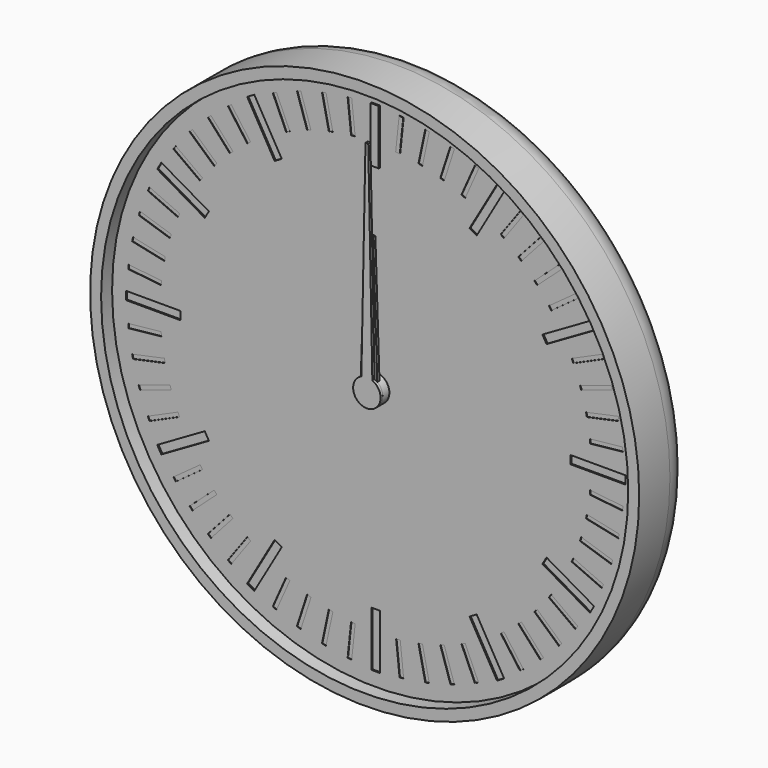
from build123d import *

# Parameters (mm, degrees)
F0_R      = 100
F1_DEPTH  = 24
F2_R      = 10
F3_T      = -4
F4_R      = 5
F4_R_2    = 3
F5_DEPTH  = 2
F6_DEPTH  = 19
F7_DEPTH  = 8
F9_DEPTH  = 4
F11_DEPTH = 4
F12_R     = 5
F12_R_2   = 3
F13_DEPTH = 2
F14_R     = 3
F15_DEPTH = 4
F17_DEPTH = 4
F18_R     = 3
F19_DEPTH = 2
F20_R     = 98
F20_R_2   = 5
F21_DEPTH = 1
F23_R     = 5
F23_R_2   = 3
F24_DEPTH = 2
F25_W     = 3
F25_H     = 20
F25_W_2   = 20
F25_H_2   = 3
F26_DEPTH = 0.5
F27_W     = 1.5
F27_H     = 12
F27_W_2   = 12
F27_H_2   = 1.5
F28_DEPTH = 0.2
F29_DEPTH = 1
F30_DEPTH = 0.4
F31_R     = 5
F31_R_2   = 3
F32_DEPTH = 5
F33_R     = 3
F34_DEPTH = 1
F36_DEPTH = 1


with BuildPart() as f1:
    # F0 (on Front) → F1 (new body)
    with BuildSketch(Plane.XZ):
        Circle(F0_R)
    extrude(amount=F1_DEPTH)

    # F2
    f2_edges = [f1.edges().sort_by_distance(p)[0] for p in [
        (-100, 0, 0),
    ]]
    fillet(f2_edges, radius=F2_R)

    # F3
    f3_openings = [f1.faces().sort_by_distance(p)[0] for p in [
        (0, -24, 0),
    ]]
    offset(amount=F3_T, openings=f3_openings)

    # F4 (on face) → F5 (join)
    with BuildSketch(Plane.XZ.offset(4)):
        Circle(F4_R)
        Circle(F4_R_2, mode=Mode.SUBTRACT)
        with Locations((40, 0)):
            Circle(F4_R)
        with Locations((40, 0)):
            Circle(F4_R_2, mode=Mode.SUBTRACT)
    extrude(amount=F5_DEPTH)


with BuildPart() as f6:
    # F4 (on face) → F6 (new body)
    with BuildSketch(Plane.XZ.offset(4)):
        Circle(F4_R_2)
    extrude(amount=F6_DEPTH)

    # F8 (on face) → F9 (join)
    with BuildSketch(Plane.XZ.offset(6)):
        with BuildLine():
            ThreePointArc((9.2729637667, -1.3794085621), (9.3494561423, -0.6915886375), (9.375, 0))
            ThreePointArc((9.375, 0), (9.3494561423, 0.6915886375), (9.2729637667, 1.3794085621))
            ThreePointArc((9.2729637667, 1.3794085621), (8.9161548403, 2.8970343223), (8.3127812852, 4.3345463782))
            ThreePointArc((8.3127812852, 4.3345463782), (7.5845343223, 5.5104867402), (6.6911892658, 6.566476316))
            ThreePointArc((6.6911892658, 6.566476316), (5.5104867402, 7.5845343223), (4.1773988938, 8.3928519278))
            ThreePointArc((4.1773988938, 8.3928519278), (2.8970343223, 8.9161548403), (1.5536078905, 9.2453733036))
            ThreePointArc((1.5536078905, 9.2453733036), (0, 9.375), (-1.5536078905, 9.2453733036))
            ThreePointArc((-1.5536078905, 9.2453733036), (-2.8970343223, 8.9161548403), (-4.1773988938, 8.3928519278))
            ThreePointArc((-4.1773988938, 8.3928519278), (-5.5104867402, 7.5845343223), (-6.6911892658, 6.566476316))
            ThreePointArc((-6.6911892658, 6.566476316), (-7.5845343223, 5.5104867402), (-8.3127812852, 4.3345463782))
            ThreePointArc((-8.3127812852, 4.3345463782), (-8.9161548403, 2.8970343223), (-9.2729637667, 1.3794085621))
            ThreePointArc((-9.2729637667, 1.3794085621), (-9.375, 0), (-9.2729637667, -1.3794085621))
            ThreePointArc((-9.2729637667, -1.3794085621), (-8.9161548403, -2.8970343223), (-8.3127812852, -4.3345463782))
            ThreePointArc((-8.3127812852, -4.3345463782), (-7.5845343223, -5.5104867402), (-6.6911892658, -6.566476316))
            ThreePointArc((-6.6911892658, -6.566476316), (-5.5104867402, -7.5845343223), (-4.1773988938, -8.3928519278))
            ThreePointArc((-4.1773988938, -8.3928519278), (-2.8970343223, -8.9161548403), (-1.5536078905, -9.2453733036))
            ThreePointArc((-1.5536078905, -9.2453733036), (0, -9.375), (1.5536078905, -9.2453733036))
            ThreePointArc((1.5536078905, -9.2453733036), (2.8970343223, -8.9161548403), (4.1773988938, -8.3928519278))
            ThreePointArc((4.1773988938, -8.3928519278), (5.5104867402, -7.5845343223), (6.6911892658, -6.566476316))
            ThreePointArc((6.6911892658, -6.566476316), (7.5845343223, -5.5104867402), (8.3127812852, -4.3345463782))
            ThreePointArc((8.3127812852, -4.3345463782), (8.9161548403, -2.8970343223), (9.2729637667, -1.3794085621))
        make_face()
        with BuildLine():
            ThreePointArc((8.3127812852, 4.3345463782), (8.9161548403, 2.8970343223), (9.2729637667, 1.3794085621))
            Line((9.2729637667, 1.3794085621), (11.1823199426, 2.3946312492))
            Line((11.1823199426, 2.3946312492), (10.8182678729, 3.515068311))
            Line((10.8182678729, 3.515068311), (10.4542158031, 4.6355053728))
            Line((10.4542158031, 4.6355053728), (8.3127812852, 4.3345463782))
        make_face()
        with BuildLine():
            Line((11.1823199426, -2.3946312492), (9.2729637667, -1.3794085621))
            ThreePointArc((9.2729637667, -1.3794085621), (8.9161548403, -2.8970343223), (8.3127812852, -4.3345463782))
            Line((8.3127812852, -4.3345463782), (10.4542158031, -4.6355053728))
            Line((10.4542158031, -4.6355053728), (10.8182678729, -3.515068311))
            Line((10.8182678729, -3.515068311), (11.1823199426, -2.3946312492))
        make_face()
        with BuildLine():
            ThreePointArc((4.1773988938, 8.3928519278), (5.5104867402, 7.5845343223), (6.6911892658, 6.566476316))
            Line((6.6911892658, 6.566476316), (7.6391579371, 8.5101001246))
            Line((7.6391579371, 8.5101001246), (6.6860572448, 9.202568311))
            Line((6.6860572448, 9.202568311), (5.7329565525, 9.8950364974))
            Line((5.7329565525, 9.8950364974), (4.1773988938, 8.3928519278))
        make_face()
        with BuildLine():
            Line((7.6391579371, -8.5101001246), (6.6911892658, -6.566476316))
            ThreePointArc((6.6911892658, -6.566476316), (5.5104867402, -7.5845343223), (4.1773988938, -8.3928519278))
            Line((4.1773988938, -8.3928519278), (5.7329565525, -9.8950364974))
            Line((5.7329565525, -9.8950364974), (6.6860572448, -9.202568311))
            Line((6.6860572448, -9.202568311), (7.6391579371, -8.5101001246))
        make_face()
        with BuildLine():
            ThreePointArc((-1.5536078905, 9.2453733036), (0, 9.375), (1.5536078905, 9.2453733036))
            Line((1.5536078905, 9.2453733036), (1.1780972451, 11.375))
            Line((1.1780972451, 11.375), (0, 11.375))
            Line((0, 11.375), (-1.1780972451, 11.375))
            Line((-1.1780972451, 11.375), (-1.5536078905, 9.2453733036))
        make_face()
        with BuildLine():
            Line((1.1780972451, -11.375), (1.5536078905, -9.2453733036))
            ThreePointArc((1.5536078905, -9.2453733036), (0, -9.375), (-1.5536078905, -9.2453733036))
            Line((-1.5536078905, -9.2453733036), (-1.1780972451, -11.375))
            Line((-1.1780972451, -11.375), (0, -11.375))
            Line((0, -11.375), (1.1780972451, -11.375))
        make_face()
        with BuildLine():
            ThreePointArc((-6.6911892658, 6.566476316), (-5.5104867402, 7.5845343223), (-4.1773988938, 8.3928519278))
            Line((-4.1773988938, 8.3928519278), (-5.7329565525, 9.8950364974))
            Line((-5.7329565525, 9.8950364974), (-6.6860572448, 9.202568311))
            Line((-6.6860572448, 9.202568311), (-7.6391579371, 8.5101001246))
            Line((-7.6391579371, 8.5101001246), (-6.6911892658, 6.566476316))
        make_face()
        with BuildLine():
            Line((-5.7329565525, -9.8950364974), (-4.1773988938, -8.3928519278))
            ThreePointArc((-4.1773988938, -8.3928519278), (-5.5104867402, -7.5845343223), (-6.6911892658, -6.566476316))
            Line((-6.6911892658, -6.566476316), (-7.6391579371, -8.5101001246))
            Line((-7.6391579371, -8.5101001246), (-6.6860572448, -9.202568311))
            Line((-6.6860572448, -9.202568311), (-5.7329565525, -9.8950364974))
        make_face()
        with BuildLine():
            ThreePointArc((-9.2729637667, 1.3794085621), (-8.9161548403, 2.8970343223), (-8.3127812852, 4.3345463782))
            Line((-8.3127812852, 4.3345463782), (-10.4542158031, 4.6355053728))
            Line((-10.4542158031, 4.6355053728), (-10.8182678729, 3.515068311))
            Line((-10.8182678729, 3.515068311), (-11.1823199426, 2.3946312492))
            Line((-11.1823199426, 2.3946312492), (-9.2729637667, 1.3794085621))
        make_face()
        with BuildLine():
            Line((-10.4542158031, -4.6355053728), (-8.3127812852, -4.3345463782))
            ThreePointArc((-8.3127812852, -4.3345463782), (-8.9161548403, -2.8970343223), (-9.2729637667, -1.3794085621))
            Line((-9.2729637667, -1.3794085621), (-11.1823199426, -2.3946312492))
            Line((-11.1823199426, -2.3946312492), (-10.8182678729, -3.515068311))
            Line((-10.8182678729, -3.515068311), (-10.4542158031, -4.6355053728))
        make_face()
    extrude(amount=F9_DEPTH)

    # F35 (on face) → F36 (join)
    with BuildSketch(Plane.XZ.offset(23)):
        with BuildLine():
            ThreePointArc((-2, 4.582575695), (-2.7386127875, -4.1833001327), (5, 0))
            ThreePointArc((5, 0), (4.1833001327, 2.7386127875), (2, 4.582575695))
            ThreePointArc((2, 4.582575695), (0, 5), (-2, 4.582575695))
        make_face()
        with BuildLine():
            ThreePointArc((-2, 4.582575695), (0, 5), (2, 4.582575695))
            Line((2, 4.582575695), (0.5, 80))
            Line((0.5, 80), (0, 80))
            Line((0, 80), (-0.5, 80))
            Line((-0.5, 80), (-2, 4.582575695))
        make_face()
    extrude(amount=-F36_DEPTH)


with BuildPart() as f7:
    # F4 (on face) → F7 (new body)
    with BuildSketch(Plane.XZ.offset(4)):
        with Locations((40, 0)):
            Circle(F4_R_2)
    extrude(amount=F7_DEPTH)

    # F10 (on face) → F11 (join)
    with BuildSketch(Plane.XZ.offset(6)):
        with BuildLine():
            ThreePointArc((68.0829066802, -1.5381733945), (68.1144747006, -0.7693746225), (68.125, 0))
            ThreePointArc((68.125, 0), (68.1144747006, 0.7693746225), (68.0829066802, 1.5381733945))
            ThreePointArc((68.0829066802, 1.5381733945), (67.9709283072, 2.9398630294), (67.7890320221, 4.3342039956))
            ThreePointArc((67.7890320221, 4.3342039956), (67.5104012706, 5.8475163042), (67.1494235596, 7.3433252263))
            ThreePointArc((67.1494235596, 7.3433252263), (66.7484645208, 8.6911029668), (66.280643318, 10.0171558733))
            ThreePointArc((66.280643318, 10.0171558733), (65.6934659962, 11.4394680865), (65.0293803521, 12.8275385085))
            ThreePointArc((65.0293803521, 12.8275385085), (64.3569644814, 14.0625), (63.6236643925, 15.2623099717))
            ThreePointArc((63.6236643925, 15.2623099717), (62.7536029668, 16.5314602207), (61.815433119, 17.7511268046))
            ThreePointArc((61.815433119, 17.7511268046), (60.9009482166, 18.8192983038), (59.934217974, 19.8404278876))
            ThreePointArc((59.934217974, 19.8404278876), (58.8192983038, 20.9009482166), (57.6480467764, 21.8989056799))
            ThreePointArc((57.6480467764, 21.8989056799), (56.5314602207, 22.7536029668), (55.3735505752, 23.5514238999))
            ThreePointArc((55.3735505752, 23.5514238999), (54.0625, 24.3569644814), (52.709356105, 25.0895972944))
            ThreePointArc((52.709356105, 25.0895972944), (51.4394680865, 25.6934659962), (50.1409852457, 26.2331096755))
            ThreePointArc((50.1409852457, 26.2331096755), (48.6911029668, 26.7484645208), (47.2152055856, 27.1837531139))
            ThreePointArc((47.2152055856, 27.1837531139), (45.8475163042, 27.5104012706), (44.4652101991, 27.7682826779))
            ThreePointArc((44.4652101991, 27.7682826779), (42.9398630294, 27.9709283072), (41.4057159597, 28.0898484802))
            ThreePointArc((41.4057159597, 28.0898484802), (40, 28.125), (38.5942840403, 28.0898484802))
            ThreePointArc((38.5942840403, 28.0898484802), (37.0601369706, 27.9709283072), (35.5347898009, 27.7682826779))
            ThreePointArc((35.5347898009, 27.7682826779), (34.1524836958, 27.5104012706), (32.7847944144, 27.1837531139))
            ThreePointArc((32.7847944144, 27.1837531139), (31.3088970332, 26.7484645208), (29.8590147543, 26.2331096755))
            ThreePointArc((29.8590147543, 26.2331096755), (28.5605319135, 25.6934659962), (27.290643895, 25.0895972944))
            ThreePointArc((27.290643895, 25.0895972944), (25.9375, 24.3569644814), (24.6264494248, 23.5514238999))
            ThreePointArc((24.6264494248, 23.5514238999), (23.4685397793, 22.7536029668), (22.3519532236, 21.8989056799))
            ThreePointArc((22.3519532236, 21.8989056799), (21.1807016962, 20.9009482166), (20.065782026, 19.8404278876))
            ThreePointArc((20.065782026, 19.8404278876), (19.0990517834, 18.8192983038), (18.184566881, 17.7511268046))
            ThreePointArc((18.184566881, 17.7511268046), (17.2463970332, 16.5314602207), (16.3763356075, 15.2623099717))
            ThreePointArc((16.3763356075, 15.2623099717), (15.6430355186, 14.0625), (14.9706196479, 12.8275385085))
            ThreePointArc((14.9706196479, 12.8275385085), (14.3065340038, 11.4394680865), (13.719356682, 10.0171558733))
            ThreePointArc((13.719356682, 10.0171558733), (13.2515354792, 8.6911029668), (12.8505764404, 7.3433252263))
            ThreePointArc((12.8505764404, 7.3433252263), (12.4895987294, 5.8475163042), (12.2109679779, 4.3342039956))
            ThreePointArc((12.2109679779, 4.3342039956), (12.0290716928, 2.9398630294), (11.9170933198, 1.5381733945))
            ThreePointArc((11.9170933198, 1.5381733945), (11.875, 0), (11.9170933198, -1.5381733945))
            ThreePointArc((11.9170933198, -1.5381733945), (12.0290716928, -2.9398630294), (12.2109679779, -4.3342039956))
            ThreePointArc((12.2109679779, -4.3342039956), (12.4895987294, -5.8475163042), (12.8505764404, -7.3433252263))
            ThreePointArc((12.8505764404, -7.3433252263), (13.2515354792, -8.6911029668), (13.719356682, -10.0171558733))
            ThreePointArc((13.719356682, -10.0171558733), (14.3065340038, -11.4394680865), (14.9706196479, -12.8275385085))
            ThreePointArc((14.9706196479, -12.8275385085), (15.6430355186, -14.0625), (16.3763356075, -15.2623099717))
            ThreePointArc((16.3763356075, -15.2623099717), (17.2463970332, -16.5314602207), (18.184566881, -17.7511268046))
            ThreePointArc((18.184566881, -17.7511268046), (19.0990517834, -18.8192983038), (20.065782026, -19.8404278876))
            ThreePointArc((20.065782026, -19.8404278876), (21.1807016962, -20.9009482166), (22.3519532236, -21.8989056799))
            ThreePointArc((22.3519532236, -21.8989056799), (23.4685397793, -22.7536029668), (24.6264494248, -23.5514238999))
            ThreePointArc((24.6264494248, -23.5514238999), (25.9375, -24.3569644814), (27.290643895, -25.0895972944))
            ThreePointArc((27.290643895, -25.0895972944), (28.5605319135, -25.6934659962), (29.8590147543, -26.2331096755))
            ThreePointArc((29.8590147543, -26.2331096755), (31.3088970332, -26.7484645208), (32.7847944144, -27.1837531139))
            ThreePointArc((32.7847944144, -27.1837531139), (34.1524836958, -27.5104012706), (35.5347898009, -27.7682826779))
            ThreePointArc((35.5347898009, -27.7682826779), (37.0601369706, -27.9709283072), (38.5942840403, -28.0898484802))
            ThreePointArc((38.5942840403, -28.0898484802), (40, -28.125), (41.4057159597, -28.0898484802))
            ThreePointArc((41.4057159597, -28.0898484802), (42.9398630294, -27.9709283072), (44.4652101991, -27.7682826779))
            ThreePointArc((44.4652101991, -27.7682826779), (45.8475163042, -27.5104012706), (47.2152055856, -27.1837531139))
            ThreePointArc((47.2152055856, -27.1837531139), (48.6911029668, -26.7484645208), (50.1409852457, -26.2331096755))
            ThreePointArc((50.1409852457, -26.2331096755), (51.4394680865, -25.6934659962), (52.709356105, -25.0895972944))
            ThreePointArc((52.709356105, -25.0895972944), (54.0625, -24.3569644814), (55.3735505752, -23.5514238999))
            ThreePointArc((55.3735505752, -23.5514238999), (56.5314602207, -22.7536029668), (57.6480467764, -21.8989056799))
            ThreePointArc((57.6480467764, -21.8989056799), (58.8192983038, -20.9009482166), (59.934217974, -19.8404278876))
            ThreePointArc((59.934217974, -19.8404278876), (60.9009482166, -18.8192983038), (61.815433119, -17.7511268046))
            ThreePointArc((61.815433119, -17.7511268046), (62.7536029668, -16.5314602207), (63.6236643925, -15.2623099717))
            ThreePointArc((63.6236643925, -15.2623099717), (64.3569644814, -14.0625), (65.0293803521, -12.8275385085))
            ThreePointArc((65.0293803521, -12.8275385085), (65.6934659962, -11.4394680865), (66.280643318, -10.0171558733))
            ThreePointArc((66.280643318, -10.0171558733), (66.7484645208, -8.6911029668), (67.1494235596, -7.3433252263))
            ThreePointArc((67.1494235596, -7.3433252263), (67.5104012706, -5.8475163042), (67.7890320221, -4.3342039956))
            ThreePointArc((67.7890320221, -4.3342039956), (67.9709283072, -2.9398630294), (68.0829066802, -1.5381733945))
        make_face()
        with BuildLine():
            ThreePointArc((68.0829066802, 1.5381733945), (68.1144747006, 0.7693746225), (68.125, 0))
            ThreePointArc((68.125, 0), (68.1144747006, -0.7693746225), (68.0829066802, -1.5381733945))
            Line((68.0829066802, -1.5381733945), (70.125, -1.1780972451))
            Line((70.125, -1.1780972451), (70.125, 0))
            Line((70.125, 0), (70.125, 1.1780972451))
            Line((70.125, 1.1780972451), (68.0829066802, 1.5381733945))
        make_face()
        with BuildLine():
            ThreePointArc((67.1494235596, 7.3433252263), (67.5104012706, 5.8475163042), (67.7890320221, 4.3342039956))
            Line((67.7890320221, 4.3342039956), (69.7116366623, 5.1109866922))
            Line((69.7116366623, 5.1109866922), (69.4666964721, 6.2633396859))
            Line((69.4666964721, 6.2633396859), (69.2217562819, 7.4156926796))
            Line((69.2217562819, 7.4156926796), (67.1494235596, 7.3433252263))
        make_face()
        with BuildLine():
            Line((69.7116366623, -5.1109866922), (67.7890320221, -4.3342039956))
            ThreePointArc((67.7890320221, -4.3342039956), (67.5104012706, -5.8475163042), (67.1494235596, -7.3433252263))
            Line((67.1494235596, -7.3433252263), (69.2217562819, -7.4156926796))
            Line((69.2217562819, -7.4156926796), (69.4666964721, -6.2633396859))
            Line((69.4666964721, -6.2633396859), (69.7116366623, -5.1109866922))
        make_face()
        with BuildLine():
            ThreePointArc((65.0293803521, 12.8275385085), (65.6934659962, 11.4394680865), (66.280643318, 10.0171558733))
            Line((66.280643318, 10.0171558733), (67.9997322302, 11.1766959857))
            Line((67.9997322302, 11.1766959857), (67.5205569115, 12.2529413727))
            Line((67.5205569115, 12.2529413727), (67.0413815928, 13.3291867596))
            Line((67.0413815928, 13.3291867596), (65.0293803521, 12.8275385085))
        make_face()
        with BuildLine():
            Line((67.9997322302, -11.1766959857), (66.280643318, -10.0171558733))
            ThreePointArc((66.280643318, -10.0171558733), (65.6934659962, -11.4394680865), (65.0293803521, -12.8275385085))
            Line((65.0293803521, -12.8275385085), (67.0413815928, -13.3291867596))
            Line((67.0413815928, -13.3291867596), (67.5205569115, -12.2529413727))
            Line((67.5205569115, -12.2529413727), (67.9997322302, -11.1766959857))
        make_face()
        with BuildLine():
            ThreePointArc((61.815433119, 17.7511268046), (62.7536029668, 16.5314602207), (63.6236643925, 15.2623099717))
            Line((63.6236643925, 15.2623099717), (65.064105142, 16.753930033))
            Line((65.064105142, 16.753930033), (64.3716369555, 17.7070307253))
            Line((64.3716369555, 17.7070307253), (63.6791687691, 18.6601314176))
            Line((63.6791687691, 18.6601314176), (61.815433119, 17.7511268046))
        make_face()
        with BuildLine():
            Line((65.064105142, -16.753930033), (63.6236643925, -15.2623099717))
            ThreePointArc((63.6236643925, -15.2623099717), (62.7536029668, -16.5314602207), (61.815433119, -17.7511268046))
            Line((61.815433119, -17.7511268046), (63.6791687691, -18.6601314176))
            Line((63.6791687691, -18.6601314176), (64.3716369555, -17.7070307253))
            Line((64.3716369555, -17.7070307253), (65.064105142, -16.753930033))
        make_face()
        with BuildLine():
            ThreePointArc((57.6480467764, 21.8989056799), (58.8192983038, 20.9009482166), (59.934217974, 19.8404278876))
            Line((59.934217974, 19.8404278876), (61.0330563882, 21.5989369435))
            Line((61.0330563882, 21.5989369435), (60.1575595166, 22.3872378675))
            Line((60.1575595166, 22.3872378675), (59.282062645, 23.1755387915))
            Line((59.282062645, 23.1755387915), (57.6480467764, 21.8989056799))
        make_face()
        with BuildLine():
            Line((61.0330563882, -21.5989369435), (59.934217974, -19.8404278876))
            ThreePointArc((59.934217974, -19.8404278876), (58.8192983038, -20.9009482166), (57.6480467764, -21.8989056799))
            Line((57.6480467764, -21.8989056799), (59.282062645, -23.1755387915))
            Line((59.282062645, -23.1755387915), (60.1575595166, -22.3872378675))
            Line((60.1575595166, -22.3872378675), (61.0330563882, -21.5989369435))
        make_face()
        with BuildLine():
            ThreePointArc((52.709356105, 25.0895972944), (54.0625, 24.3569644814), (55.3735505752, 23.5514238999))
            Line((55.3735505752, 23.5514238999), (56.0827621424, 25.4999666665))
            Line((56.0827621424, 25.4999666665), (55.0625, 26.089015289))
            Line((55.0625, 26.089015289), (54.0422378576, 26.6780639116))
            Line((54.0422378576, 26.6780639116), (52.709356105, 25.0895972944))
        make_face()
        with BuildLine():
            Line((56.0827621424, -25.4999666665), (55.3735505752, -23.5514238999))
            ThreePointArc((55.3735505752, -23.5514238999), (54.0625, -24.3569644814), (52.709356105, -25.0895972944))
            Line((52.709356105, -25.0895972944), (54.0422378576, -26.6780639116))
            Line((54.0422378576, -26.6780639116), (55.0625, -26.089015289))
            Line((55.0625, -26.089015289), (56.0827621424, -25.4999666665))
        make_face()
        with BuildLine():
            ThreePointArc((47.2152055856, 27.1837531139), (48.6911029668, 26.7484645208), (50.1409852457, 26.2331096755))
            Line((50.1409852457, 26.2331096755), (50.4295740173, 28.2865254836))
            Line((50.4295740173, 28.2865254836), (49.3091369555, 28.6505775534))
            Line((49.3091369555, 28.6505775534), (48.1886998938, 29.0146296232))
            Line((48.1886998938, 29.0146296232), (47.2152055856, 27.1837531139))
        make_face()
        with BuildLine():
            Line((50.4295740173, -28.2865254836), (50.1409852457, -26.2331096755))
            ThreePointArc((50.1409852457, -26.2331096755), (48.6911029668, -26.7484645208), (47.2152055856, -27.1837531139))
            Line((47.2152055856, -27.1837531139), (48.1886998938, -29.0146296232))
            Line((48.1886998938, -29.0146296232), (49.3091369555, -28.6505775534))
            Line((49.3091369555, -28.6505775534), (50.4295740173, -28.2865254836))
        make_face()
        with BuildLine():
            ThreePointArc((41.4057159597, 28.0898484802), (42.9398630294, 27.9709283072), (44.4652101991, 27.7682826779))
            Line((44.4652101991, 27.7682826779), (44.3205634611, 29.8368274034))
            Line((44.3205634611, 29.8368274034), (43.1489199559, 29.959972098))
            Line((43.1489199559, 29.959972098), (41.9772764508, 30.0831167926))
            Line((41.9772764508, 30.0831167926), (41.4057159597, 28.0898484802))
        make_face()
        with BuildLine():
            Line((44.3205634611, -29.8368274034), (44.4652101991, -27.7682826779))
            ThreePointArc((44.4652101991, -27.7682826779), (42.9398630294, -27.9709283072), (41.4057159597, -28.0898484802))
            Line((41.4057159597, -28.0898484802), (41.9772764508, -30.0831167926))
            Line((41.9772764508, -30.0831167926), (43.1489199559, -29.959972098))
            Line((43.1489199559, -29.959972098), (44.3205634611, -29.8368274034))
        make_face()
        with BuildLine():
            ThreePointArc((35.5347898009, 27.7682826779), (37.0601369706, 27.9709283072), (38.5942840403, 28.0898484802))
            Line((38.5942840403, 28.0898484802), (38.0227235492, 30.0831167926))
            Line((38.0227235492, 30.0831167926), (36.8510800441, 29.959972098))
            Line((36.8510800441, 29.959972098), (35.6794365389, 29.8368274034))
            Line((35.6794365389, 29.8368274034), (35.5347898009, 27.7682826779))
        make_face()
        with BuildLine():
            Line((38.0227235492, -30.0831167926), (38.5942840403, -28.0898484802))
            ThreePointArc((38.5942840403, -28.0898484802), (37.0601369706, -27.9709283072), (35.5347898009, -27.7682826779))
            Line((35.5347898009, -27.7682826779), (35.6794365389, -29.8368274034))
            Line((35.6794365389, -29.8368274034), (36.8510800441, -29.959972098))
            Line((36.8510800441, -29.959972098), (38.0227235492, -30.0831167926))
        make_face()
        with BuildLine():
            ThreePointArc((29.8590147543, 26.2331096755), (31.3088970332, 26.7484645208), (32.7847944144, 27.1837531139))
            Line((32.7847944144, 27.1837531139), (31.8113001062, 29.0146296232))
            Line((31.8113001062, 29.0146296232), (30.6908630445, 28.6505775534))
            Line((30.6908630445, 28.6505775534), (29.5704259827, 28.2865254836))
            Line((29.5704259827, 28.2865254836), (29.8590147543, 26.2331096755))
        make_face()
        with BuildLine():
            Line((31.8113001062, -29.0146296232), (32.7847944144, -27.1837531139))
            ThreePointArc((32.7847944144, -27.1837531139), (31.3088970332, -26.7484645208), (29.8590147543, -26.2331096755))
            Line((29.8590147543, -26.2331096755), (29.5704259827, -28.2865254836))
            Line((29.5704259827, -28.2865254836), (30.6908630445, -28.6505775534))
            Line((30.6908630445, -28.6505775534), (31.8113001062, -29.0146296232))
        make_face()
        with BuildLine():
            ThreePointArc((24.6264494248, 23.5514238999), (25.9375, 24.3569644814), (27.290643895, 25.0895972944))
            Line((27.290643895, 25.0895972944), (25.9577621424, 26.6780639116))
            Line((25.9577621424, 26.6780639116), (24.9375, 26.089015289))
            Line((24.9375, 26.089015289), (23.9172378576, 25.4999666665))
            Line((23.9172378576, 25.4999666665), (24.6264494248, 23.5514238999))
        make_face()
        with BuildLine():
            Line((25.9577621424, -26.6780639116), (27.290643895, -25.0895972944))
            ThreePointArc((27.290643895, -25.0895972944), (25.9375, -24.3569644814), (24.6264494248, -23.5514238999))
            Line((24.6264494248, -23.5514238999), (23.9172378576, -25.4999666665))
            Line((23.9172378576, -25.4999666665), (24.9375, -26.089015289))
            Line((24.9375, -26.089015289), (25.9577621424, -26.6780639116))
        make_face()
        with BuildLine():
            ThreePointArc((20.065782026, 19.8404278876), (21.1807016962, 20.9009482166), (22.3519532236, 21.8989056799))
            Line((22.3519532236, 21.8989056799), (20.717937355, 23.1755387915))
            Line((20.717937355, 23.1755387915), (19.8424404834, 22.3872378675))
            Line((19.8424404834, 22.3872378675), (18.9669436118, 21.5989369435))
            Line((18.9669436118, 21.5989369435), (20.065782026, 19.8404278876))
        make_face()
        with BuildLine():
            Line((20.717937355, -23.1755387915), (22.3519532236, -21.8989056799))
            ThreePointArc((22.3519532236, -21.8989056799), (21.1807016962, -20.9009482166), (20.065782026, -19.8404278876))
            Line((20.065782026, -19.8404278876), (18.9669436118, -21.5989369435))
            Line((18.9669436118, -21.5989369435), (19.8424404834, -22.3872378675))
            Line((19.8424404834, -22.3872378675), (20.717937355, -23.1755387915))
        make_face()
        with BuildLine():
            ThreePointArc((16.3763356075, 15.2623099717), (17.2463970332, 16.5314602207), (18.184566881, 17.7511268046))
            Line((18.184566881, 17.7511268046), (16.3208312309, 18.6601314176))
            Line((16.3208312309, 18.6601314176), (15.6283630445, 17.7070307253))
            Line((15.6283630445, 17.7070307253), (14.935894858, 16.753930033))
            Line((14.935894858, 16.753930033), (16.3763356075, 15.2623099717))
        make_face()
        with BuildLine():
            Line((16.3208312309, -18.6601314176), (18.184566881, -17.7511268046))
            ThreePointArc((18.184566881, -17.7511268046), (17.2463970332, -16.5314602207), (16.3763356075, -15.2623099717))
            Line((16.3763356075, -15.2623099717), (14.935894858, -16.753930033))
            Line((14.935894858, -16.753930033), (15.6283630445, -17.7070307253))
            Line((15.6283630445, -17.7070307253), (16.3208312309, -18.6601314176))
        make_face()
        with BuildLine():
            ThreePointArc((13.719356682, 10.0171558733), (14.3065340038, 11.4394680865), (14.9706196479, 12.8275385085))
            Line((14.9706196479, 12.8275385085), (12.9586184072, 13.3291867596))
            Line((12.9586184072, 13.3291867596), (12.4794430885, 12.2529413727))
            Line((12.4794430885, 12.2529413727), (12.0002677698, 11.1766959857))
            Line((12.0002677698, 11.1766959857), (13.719356682, 10.0171558733))
        make_face()
        with BuildLine():
            Line((12.9586184072, -13.3291867596), (14.9706196479, -12.8275385085))
            ThreePointArc((14.9706196479, -12.8275385085), (14.3065340038, -11.4394680865), (13.719356682, -10.0171558733))
            Line((13.719356682, -10.0171558733), (12.0002677698, -11.1766959857))
            Line((12.0002677698, -11.1766959857), (12.4794430885, -12.2529413727))
            Line((12.4794430885, -12.2529413727), (12.9586184072, -13.3291867596))
        make_face()
        with BuildLine():
            ThreePointArc((12.2109679779, 4.3342039956), (12.4895987294, 5.8475163042), (12.8505764404, 7.3433252263))
            Line((12.8505764404, 7.3433252263), (10.7782437181, 7.4156926796))
            Line((10.7782437181, 7.4156926796), (10.5333035279, 6.2633396859))
            Line((10.5333035279, 6.2633396859), (10.2883633377, 5.1109866922))
            Line((10.2883633377, 5.1109866922), (12.2109679779, 4.3342039956))
        make_face()
        with BuildLine():
            Line((10.7782437181, -7.4156926796), (12.8505764404, -7.3433252263))
            ThreePointArc((12.8505764404, -7.3433252263), (12.4895987294, -5.8475163042), (12.2109679779, -4.3342039956))
            Line((12.2109679779, -4.3342039956), (10.2883633377, -5.1109866922))
            Line((10.2883633377, -5.1109866922), (10.5333035279, -6.2633396859))
            Line((10.5333035279, -6.2633396859), (10.7782437181, -7.4156926796))
        make_face()
        with BuildLine():
            ThreePointArc((11.9170933198, -1.5381733945), (11.875, 0), (11.9170933198, 1.5381733945))
            Line((11.9170933198, 1.5381733945), (9.875, 1.1780972451))
            Line((9.875, 1.1780972451), (9.875, 0))
            Line((9.875, 0), (9.875, -1.1780972451))
            Line((9.875, -1.1780972451), (11.9170933198, -1.5381733945))
        make_face()
    extrude(amount=F11_DEPTH)

    # F16 (on face) → F17 (join)
    with BuildSketch(Plane.XZ.offset(12)):
        with BuildLine():
            ThreePointArc((47.4288750323, -1.0304444454), (47.4821976298, -0.5164480894), (47.5, 0))
            ThreePointArc((47.5, 0), (47.4821976298, 0.5164480894), (47.4288750323, 1.0304444454))
            ThreePointArc((47.4288750323, 1.0304444454), (47.1329238722, 2.3176274578), (46.6157661985, 3.532936117))
            ThreePointArc((46.6157661985, 3.532936117), (46.0676274578, 4.4083893922), (45.4044061018, 5.2002302532))
            ThreePointArc((45.4044061018, 5.2002302532), (44.4083893922, 6.0676274578), (43.2756595386, 6.7468551628))
            ThreePointArc((43.2756595386, 6.7468551628), (42.3176274578, 7.1329238722), (41.3156377295, 7.3837048536))
            ThreePointArc((41.3156377295, 7.3837048536), (40, 7.5), (38.6843622705, 7.3837048536))
            ThreePointArc((38.6843622705, 7.3837048536), (37.6823725422, 7.1329238722), (36.7243404614, 6.7468551628))
            ThreePointArc((36.7243404614, 6.7468551628), (35.5916106078, 6.0676274578), (34.5955938982, 5.2002302532))
            ThreePointArc((34.5955938982, 5.2002302532), (33.9323725422, 4.4083893922), (33.3842338015, 3.532936117))
            ThreePointArc((33.3842338015, 3.532936117), (32.8670761278, 2.3176274578), (32.5711249677, 1.0304444454))
            ThreePointArc((32.5711249677, 1.0304444454), (32.5, 0), (32.5711249677, -1.0304444454))
            ThreePointArc((32.5711249677, -1.0304444454), (32.8670761278, -2.3176274578), (33.3842338015, -3.532936117))
            ThreePointArc((33.3842338015, -3.532936117), (33.9323725422, -4.4083893922), (34.5955938982, -5.2002302532))
            ThreePointArc((34.5955938982, -5.2002302532), (35.5916106078, -6.0676274578), (36.7243404614, -6.7468551628))
            ThreePointArc((36.7243404614, -6.7468551628), (37.6823725422, -7.1329238722), (38.6843622705, -7.3837048536))
            ThreePointArc((38.6843622705, -7.3837048536), (40, -7.5), (41.3156377295, -7.3837048536))
            ThreePointArc((41.3156377295, -7.3837048536), (42.3176274578, -7.1329238722), (43.2756595386, -6.7468551628))
            ThreePointArc((43.2756595386, -6.7468551628), (44.4083893922, -6.0676274578), (45.4044061018, -5.2002302532))
            ThreePointArc((45.4044061018, -5.2002302532), (46.0676274578, -4.4083893922), (46.6157661985, -3.532936117))
            ThreePointArc((46.6157661985, -3.532936117), (47.1329238722, -2.3176274578), (47.4288750323, -1.0304444454))
        make_face()
        with BuildLine():
            ThreePointArc((46.6157661985, 3.532936117), (47.1329238722, 2.3176274578), (47.4288750323, 1.0304444454))
            Line((47.4288750323, 1.0304444454), (49.3262785606, 2.0393117971))
            Line((49.3262785606, 2.0393117971), (48.743795249, 3.832011096))
            Line((48.743795249, 3.832011096), (46.6157661985, 3.532936117))
        make_face()
        with BuildLine():
            Line((49.3262785606, -2.0393117971), (47.4288750323, -1.0304444454))
            ThreePointArc((47.4288750323, -1.0304444454), (47.1329238722, -2.3176274578), (46.6157661985, -3.532936117))
            Line((46.6157661985, -3.532936117), (48.743795249, -3.832011096))
            Line((48.743795249, -3.832011096), (49.3262785606, -2.0393117971))
        make_face()
        with BuildLine():
            ThreePointArc((43.2756595386, 6.7468551628), (44.4083893922, 6.0676274578), (45.4044061018, 5.2002302532))
            Line((45.4044061018, 5.2002302532), (46.3464404506, 7.1316868974))
            Line((46.3464404506, 7.1316868974), (44.8214793429, 8.2396359957))
            Line((44.8214793429, 8.2396359957), (43.2756595386, 6.7468551628))
        make_face()
        with BuildLine():
            Line((46.3464404506, -7.1316868974), (45.4044061018, -5.2002302532))
            ThreePointArc((45.4044061018, -5.2002302532), (44.4083893922, -6.0676274578), (43.2756595386, -6.7468551628))
            Line((43.2756595386, -6.7468551628), (44.8214793429, -8.2396359957))
            Line((44.8214793429, -8.2396359957), (46.3464404506, -7.1316868974))
        make_face()
        with BuildLine():
            ThreePointArc((38.6843622705, 7.3837048536), (40, 7.5), (41.3156377295, 7.3837048536))
            Line((41.3156377295, 7.3837048536), (40.9424777961, 9.5))
            Line((40.9424777961, 9.5), (39.0575222039, 9.5))
            Line((39.0575222039, 9.5), (38.6843622705, 7.3837048536))
        make_face()
        with BuildLine():
            Line((40.9424777961, -9.5), (41.3156377295, -7.3837048536))
            ThreePointArc((41.3156377295, -7.3837048536), (40, -7.5), (38.6843622705, -7.3837048536))
            Line((38.6843622705, -7.3837048536), (39.0575222039, -9.5))
            Line((39.0575222039, -9.5), (40.9424777961, -9.5))
        make_face()
        with BuildLine():
            ThreePointArc((34.5955938982, 5.2002302532), (35.5916106078, 6.0676274578), (36.7243404614, 6.7468551628))
            Line((36.7243404614, 6.7468551628), (35.1785206571, 8.2396359957))
            Line((35.1785206571, 8.2396359957), (33.6535595494, 7.1316868974))
            Line((33.6535595494, 7.1316868974), (34.5955938982, 5.2002302532))
        make_face()
        with BuildLine():
            Line((35.1785206571, -8.2396359957), (36.7243404614, -6.7468551628))
            ThreePointArc((36.7243404614, -6.7468551628), (35.5916106078, -6.0676274578), (34.5955938982, -5.2002302532))
            Line((34.5955938982, -5.2002302532), (33.6535595494, -7.1316868974))
            Line((33.6535595494, -7.1316868974), (35.1785206571, -8.2396359957))
        make_face()
        with BuildLine():
            ThreePointArc((32.5711249677, 1.0304444454), (32.8670761278, 2.3176274578), (33.3842338015, 3.532936117))
            Line((33.3842338015, 3.532936117), (31.256204751, 3.832011096))
            Line((31.256204751, 3.832011096), (30.6737214394, 2.0393117971))
            Line((30.6737214394, 2.0393117971), (32.5711249677, 1.0304444454))
        make_face()
        with BuildLine():
            Line((31.256204751, -3.832011096), (33.3842338015, -3.532936117))
            ThreePointArc((33.3842338015, -3.532936117), (32.8670761278, -2.3176274578), (32.5711249677, -1.0304444454))
            Line((32.5711249677, -1.0304444454), (30.6737214394, -2.0393117971))
            Line((30.6737214394, -2.0393117971), (31.256204751, -3.832011096))
        make_face()
    extrude(amount=F17_DEPTH)

    # F18 (on face) → F19 (join)
    with BuildSketch(Plane.XZ.offset(16)):
        with Locations((40, 0)):
            Circle(F18_R)
    extrude(amount=F19_DEPTH)


with BuildPart() as f13:
    # F12 (on face) → F13 (new body)
    with BuildSketch(Plane.XZ.offset(10)):
        Circle(F12_R)
        Circle(F12_R_2, mode=Mode.SUBTRACT)
    extrude(amount=F13_DEPTH)

    # F14 (on face) → F15 (join)
    with BuildSketch(Plane.XZ.offset(12)):
        with BuildLine():
            ThreePointArc((29.9718156995, -1.3001014101), (29.9929530972, -0.6502034357), (30, 0))
            ThreePointArc((30, 0), (29.9929530972, 0.6502034357), (29.9718156995, 1.3001014101))
            ThreePointArc((29.9718156995, 1.3001014101), (29.907520012, 2.3537728718), (29.8061935814, 3.4045299509))
            ThreePointArc((29.8061935814, 3.4045299509), (29.6306502179, 4.6930339512), (29.3994322443, 5.9727199596))
            ThreePointArc((29.3994322443, 5.9727199596), (29.1710976119, 7.0033609157), (28.9066440563, 8.0253304855))
            ThreePointArc((28.9066440563, 8.0253304855), (28.5316954889, 9.2705098312), (28.1031371961, 10.4982703213))
            ThreePointArc((28.1031371961, 10.4982703213), (27.7163859753, 11.480502971), (27.2953170189, 12.448520749))
            ThreePointArc((27.2953170189, 12.448520749), (26.7301957257, 13.6197149922), (26.1148496411, 14.765318426))
            ThreePointArc((26.1148496411, 14.765318426), (25.5792049306, 15.6749569415), (25.0118886885, 16.5651871174))
            ThreePointArc((25.0118886885, 16.5651871174), (24.2705098312, 17.6335575688), (23.4835278178, 18.6687953878))
            ThreePointArc((23.4835278178, 18.6687953878), (22.812178968, 19.4834414499), (22.1125846489, 20.2739636023))
            ThreePointArc((22.1125846489, 20.2739636023), (21.2132034356, 21.2132034356), (20.2739636023, 22.1125846489))
            ThreePointArc((20.2739636023, 22.1125846489), (19.4834414499, 22.812178968), (18.6687953878, 23.4835278178))
            ThreePointArc((18.6687953878, 23.4835278178), (17.6335575688, 24.2705098312), (16.5651871174, 25.0118886885))
            ThreePointArc((16.5651871174, 25.0118886885), (15.6749569415, 25.5792049306), (14.765318426, 26.1148496411))
            ThreePointArc((14.765318426, 26.1148496411), (13.6197149922, 26.7301957257), (12.448520749, 27.2953170189))
            ThreePointArc((12.448520749, 27.2953170189), (11.480502971, 27.7163859753), (10.4982703213, 28.1031371961))
            ThreePointArc((10.4982703213, 28.1031371961), (9.2705098312, 28.5316954889), (8.0253304855, 28.9066440563))
            ThreePointArc((8.0253304855, 28.9066440563), (7.0033609157, 29.1710976119), (5.9727199596, 29.3994322443))
            ThreePointArc((5.9727199596, 29.3994322443), (4.6930339512, 29.6306502179), (3.4045299509, 29.8061935814))
            ThreePointArc((3.4045299509, 29.8061935814), (2.3537728718, 29.907520012), (1.3001014101, 29.9718156995))
            ThreePointArc((1.3001014101, 29.9718156995), (0, 30), (-1.3001014101, 29.9718156995))
            ThreePointArc((-1.3001014101, 29.9718156995), (-2.3537728718, 29.907520012), (-3.4045299509, 29.8061935814))
            ThreePointArc((-3.4045299509, 29.8061935814), (-4.6930339512, 29.6306502179), (-5.9727199596, 29.3994322443))
            ThreePointArc((-5.9727199596, 29.3994322443), (-7.0033609157, 29.1710976119), (-8.0253304855, 28.9066440563))
            ThreePointArc((-8.0253304855, 28.9066440563), (-9.2705098312, 28.5316954889), (-10.4982703213, 28.1031371961))
            ThreePointArc((-10.4982703213, 28.1031371961), (-11.480502971, 27.7163859753), (-12.448520749, 27.2953170189))
            ThreePointArc((-12.448520749, 27.2953170189), (-13.6197149922, 26.7301957257), (-14.765318426, 26.1148496411))
            ThreePointArc((-14.765318426, 26.1148496411), (-15.6749569415, 25.5792049306), (-16.5651871174, 25.0118886885))
            ThreePointArc((-16.5651871174, 25.0118886885), (-17.6335575688, 24.2705098312), (-18.6687953878, 23.4835278178))
            ThreePointArc((-18.6687953878, 23.4835278178), (-19.4834414499, 22.812178968), (-20.2739636023, 22.1125846489))
            ThreePointArc((-20.2739636023, 22.1125846489), (-21.2132034356, 21.2132034356), (-22.1125846489, 20.2739636023))
            ThreePointArc((-22.1125846489, 20.2739636023), (-22.812178968, 19.4834414499), (-23.4835278178, 18.6687953878))
            ThreePointArc((-23.4835278178, 18.6687953878), (-24.2705098312, 17.6335575688), (-25.0118886885, 16.5651871174))
            ThreePointArc((-25.0118886885, 16.5651871174), (-25.5792049306, 15.6749569415), (-26.1148496411, 14.765318426))
            ThreePointArc((-26.1148496411, 14.765318426), (-26.7301957257, 13.6197149922), (-27.2953170189, 12.448520749))
            ThreePointArc((-27.2953170189, 12.448520749), (-27.7163859753, 11.480502971), (-28.1031371961, 10.4982703213))
            ThreePointArc((-28.1031371961, 10.4982703213), (-28.5316954889, 9.2705098312), (-28.9066440563, 8.0253304855))
            ThreePointArc((-28.9066440563, 8.0253304855), (-29.1710976119, 7.0033609157), (-29.3994322443, 5.9727199596))
            ThreePointArc((-29.3994322443, 5.9727199596), (-29.6306502179, 4.6930339512), (-29.8061935814, 3.4045299509))
            ThreePointArc((-29.8061935814, 3.4045299509), (-29.907520012, 2.3537728718), (-29.9718156995, 1.3001014101))
            ThreePointArc((-29.9718156995, 1.3001014101), (-30, 0), (-29.9718156995, -1.3001014101))
            ThreePointArc((-29.9718156995, -1.3001014101), (-29.907520012, -2.3537728718), (-29.8061935814, -3.4045299509))
            ThreePointArc((-29.8061935814, -3.4045299509), (-29.6306502179, -4.6930339512), (-29.3994322443, -5.9727199596))
            ThreePointArc((-29.3994322443, -5.9727199596), (-29.1710976119, -7.0033609157), (-28.9066440563, -8.0253304855))
            ThreePointArc((-28.9066440563, -8.0253304855), (-28.5316954889, -9.2705098312), (-28.1031371961, -10.4982703213))
            ThreePointArc((-28.1031371961, -10.4982703213), (-27.7163859753, -11.480502971), (-27.2953170189, -12.448520749))
            ThreePointArc((-27.2953170189, -12.448520749), (-26.7301957257, -13.6197149922), (-26.1148496411, -14.765318426))
            ThreePointArc((-26.1148496411, -14.765318426), (-25.5792049306, -15.6749569415), (-25.0118886885, -16.5651871174))
            ThreePointArc((-25.0118886885, -16.5651871174), (-24.2705098312, -17.6335575688), (-23.4835278178, -18.6687953878))
            ThreePointArc((-23.4835278178, -18.6687953878), (-22.812178968, -19.4834414499), (-22.1125846489, -20.2739636023))
            ThreePointArc((-22.1125846489, -20.2739636023), (-21.2132034356, -21.2132034356), (-20.2739636023, -22.1125846489))
            ThreePointArc((-20.2739636023, -22.1125846489), (-19.4834414499, -22.812178968), (-18.6687953878, -23.4835278178))
            ThreePointArc((-18.6687953878, -23.4835278178), (-17.6335575688, -24.2705098312), (-16.5651871174, -25.0118886885))
            ThreePointArc((-16.5651871174, -25.0118886885), (-15.6749569415, -25.5792049306), (-14.765318426, -26.1148496411))
            ThreePointArc((-14.765318426, -26.1148496411), (-13.6197149922, -26.7301957257), (-12.448520749, -27.2953170189))
            ThreePointArc((-12.448520749, -27.2953170189), (-11.480502971, -27.7163859753), (-10.4982703213, -28.1031371961))
            ThreePointArc((-10.4982703213, -28.1031371961), (-9.2705098312, -28.5316954889), (-8.0253304855, -28.9066440563))
            ThreePointArc((-8.0253304855, -28.9066440563), (-7.0033609157, -29.1710976119), (-5.9727199596, -29.3994322443))
            ThreePointArc((-5.9727199596, -29.3994322443), (-4.6930339512, -29.6306502179), (-3.4045299509, -29.8061935814))
            ThreePointArc((-3.4045299509, -29.8061935814), (-2.3537728718, -29.907520012), (-1.3001014101, -29.9718156995))
            ThreePointArc((-1.3001014101, -29.9718156995), (0, -30), (1.3001014101, -29.9718156995))
            ThreePointArc((1.3001014101, -29.9718156995), (2.3537728718, -29.907520012), (3.4045299509, -29.8061935814))
            ThreePointArc((3.4045299509, -29.8061935814), (4.6930339512, -29.6306502179), (5.9727199596, -29.3994322443))
            ThreePointArc((5.9727199596, -29.3994322443), (7.0033609157, -29.1710976119), (8.0253304855, -28.9066440563))
            ThreePointArc((8.0253304855, -28.9066440563), (9.2705098312, -28.5316954889), (10.4982703213, -28.1031371961))
            ThreePointArc((10.4982703213, -28.1031371961), (11.480502971, -27.7163859753), (12.448520749, -27.2953170189))
            ThreePointArc((12.448520749, -27.2953170189), (13.6197149922, -26.7301957257), (14.765318426, -26.1148496411))
            ThreePointArc((14.765318426, -26.1148496411), (15.6749569415, -25.5792049306), (16.5651871174, -25.0118886885))
            ThreePointArc((16.5651871174, -25.0118886885), (17.6335575688, -24.2705098312), (18.6687953878, -23.4835278178))
            ThreePointArc((18.6687953878, -23.4835278178), (19.4834414499, -22.812178968), (20.2739636023, -22.1125846489))
            ThreePointArc((20.2739636023, -22.1125846489), (21.2132034356, -21.2132034356), (22.1125846489, -20.2739636023))
            ThreePointArc((22.1125846489, -20.2739636023), (22.812178968, -19.4834414499), (23.4835278178, -18.6687953878))
            ThreePointArc((23.4835278178, -18.6687953878), (24.2705098312, -17.6335575688), (25.0118886885, -16.5651871174))
            ThreePointArc((25.0118886885, -16.5651871174), (25.5792049306, -15.6749569415), (26.1148496411, -14.765318426))
            ThreePointArc((26.1148496411, -14.765318426), (26.7301957257, -13.6197149922), (27.2953170189, -12.448520749))
            ThreePointArc((27.2953170189, -12.448520749), (27.7163859753, -11.480502971), (28.1031371961, -10.4982703213))
            ThreePointArc((28.1031371961, -10.4982703213), (28.5316954889, -9.2705098312), (28.9066440563, -8.0253304855))
            ThreePointArc((28.9066440563, -8.0253304855), (29.1710976119, -7.0033609157), (29.3994322443, -5.9727199596))
            ThreePointArc((29.3994322443, -5.9727199596), (29.6306502179, -4.6930339512), (29.8061935814, -3.4045299509))
            ThreePointArc((29.8061935814, -3.4045299509), (29.907520012, -2.3537728718), (29.9718156995, -1.3001014101))
        make_face()
        Circle(F14_R, mode=Mode.SUBTRACT)
        with BuildLine():
            ThreePointArc((29.9718156995, 1.3001014101), (29.9929530972, 0.6502034357), (30, 0))
            ThreePointArc((30, 0), (29.9929530972, -0.6502034357), (29.9718156995, -1.3001014101))
            Line((29.9718156995, -1.3001014101), (32, -0.9424777961))
            Line((32, -0.9424777961), (32, 0))
            Line((32, 0), (32, 0.9424777961))
            Line((32, 0.9424777961), (29.9718156995, 1.3001014101))
        make_face()
        with BuildLine():
            ThreePointArc((29.3994322443, 5.9727199596), (29.6306502179, 4.6930339512), (29.8061935814, 3.4045299509))
            Line((29.8061935814, 3.4045299509), (31.7534629089, 4.0750285508))
            Line((31.7534629089, 4.0750285508), (31.606026899, 5.0059028813))
            Line((31.606026899, 5.0059028813), (31.4585908892, 5.9367772117))
            Line((31.4585908892, 5.9367772117), (29.3994322443, 5.9727199596))
        make_face()
        with BuildLine():
            Line((31.7534629089, -4.0750285508), (29.8061935814, -3.4045299509))
            ThreePointArc((29.8061935814, -3.4045299509), (29.6306502179, -4.6930339512), (29.3994322443, -5.9727199596))
            Line((29.3994322443, -5.9727199596), (31.4585908892, -5.9367772117))
            Line((31.4585908892, -5.9367772117), (31.606026899, -5.0059028813))
            Line((31.606026899, -5.0059028813), (31.7534629089, -4.0750285508))
        make_face()
        with BuildLine():
            ThreePointArc((28.1031371961, 10.4982703213), (28.5316954889, 9.2705098312), (28.9066440563, 8.0253304855))
            Line((28.9066440563, 8.0253304855), (30.7250501773, 8.9921941706))
            Line((30.7250501773, 8.9921941706), (30.4338085214, 9.88854382))
            Line((30.4338085214, 9.88854382), (30.1425668656, 10.7848934694))
            Line((30.1425668656, 10.7848934694), (28.1031371961, 10.4982703213))
        make_face()
        with BuildLine():
            Line((30.7250501773, -8.9921941706), (28.9066440563, -8.0253304855))
            ThreePointArc((28.9066440563, -8.0253304855), (28.5316954889, -9.2705098312), (28.1031371961, -10.4982703213))
            Line((28.1031371961, -10.4982703213), (30.1425668656, -10.7848934694))
            Line((30.1425668656, -10.7848934694), (30.4338085214, -9.88854382))
            Line((30.4338085214, -9.88854382), (30.7250501773, -8.9921941706))
        make_face()
        with BuildLine():
            ThreePointArc((26.1148496411, 14.765318426), (26.7301957257, 13.6197149922), (27.2953170189, 12.448520749))
            Line((27.2953170189, 12.448520749), (28.9400847397, 13.6879421265))
            Line((28.9400847397, 13.6879421265), (28.512208774, 14.5276959917))
            Line((28.512208774, 14.5276959917), (28.0843328084, 15.3674498569))
            Line((28.0843328084, 15.3674498569), (26.1148496411, 14.765318426))
        make_face()
        with BuildLine():
            Line((28.9400847397, -13.6879421265), (27.2953170189, -12.448520749))
            ThreePointArc((27.2953170189, -12.448520749), (26.7301957257, -13.6197149922), (26.1148496411, -14.765318426))
            Line((26.1148496411, -14.765318426), (28.0843328084, -15.3674498569))
            Line((28.0843328084, -15.3674498569), (28.512208774, -14.5276959917))
            Line((28.512208774, -14.5276959917), (28.9400847397, -13.6879421265))
        make_face()
        with BuildLine():
            ThreePointArc((23.4835278178, 18.6687953878), (24.2705098312, 17.6335575688), (25.0118886885, 16.5651871174))
            Line((25.0118886885, 16.5651871174), (26.4425183691, 18.0466475195))
            Line((26.4425183691, 18.0466475195), (25.88854382, 18.8091280734))
            Line((25.88854382, 18.8091280734), (25.3345692709, 19.5716086272))
            Line((25.3345692709, 19.5716086272), (23.4835278178, 18.6687953878))
        make_face()
        with BuildLine():
            Line((26.4425183691, -18.0466475195), (25.0118886885, -16.5651871174))
            ThreePointArc((25.0118886885, -16.5651871174), (24.2705098312, -17.6335575688), (23.4835278178, -18.6687953878))
            Line((23.4835278178, -18.6687953878), (25.3345692709, -19.5716086272))
            Line((25.3345692709, -19.5716086272), (25.88854382, -18.8091280734))
            Line((25.88854382, -18.8091280734), (26.4425183691, -18.0466475195))
        make_face()
        with BuildLine():
            ThreePointArc((20.2739636023, 22.1125846489), (21.2132034356, 21.2132034356), (22.1125846489, 20.2739636023))
            Line((22.1125846489, 20.2739636023), (23.2938494387, 21.9609845572))
            Line((23.2938494387, 21.9609845572), (22.627416998, 22.627416998))
            Line((22.627416998, 22.627416998), (21.9609845572, 23.2938494387))
            Line((21.9609845572, 23.2938494387), (20.2739636023, 22.1125846489))
        make_face()
        with BuildLine():
            Line((23.2938494387, -21.9609845572), (22.1125846489, -20.2739636023))
            ThreePointArc((22.1125846489, -20.2739636023), (21.2132034356, -21.2132034356), (20.2739636023, -22.1125846489))
            Line((20.2739636023, -22.1125846489), (21.9609845572, -23.2938494387))
            Line((21.9609845572, -23.2938494387), (22.627416998, -22.627416998))
            Line((22.627416998, -22.627416998), (23.2938494387, -21.9609845572))
        make_face()
        with BuildLine():
            ThreePointArc((16.5651871174, 25.0118886885), (17.6335575688, 24.2705098312), (18.6687953878, 23.4835278178))
            Line((18.6687953878, 23.4835278178), (19.5716086272, 25.3345692709))
            Line((19.5716086272, 25.3345692709), (18.8091280734, 25.88854382))
            Line((18.8091280734, 25.88854382), (18.0466475195, 26.4425183691))
            Line((18.0466475195, 26.4425183691), (16.5651871174, 25.0118886885))
        make_face()
        with BuildLine():
            Line((19.5716086272, -25.3345692709), (18.6687953878, -23.4835278178))
            ThreePointArc((18.6687953878, -23.4835278178), (17.6335575688, -24.2705098312), (16.5651871174, -25.0118886885))
            Line((16.5651871174, -25.0118886885), (18.0466475195, -26.4425183691))
            Line((18.0466475195, -26.4425183691), (18.8091280734, -25.88854382))
            Line((18.8091280734, -25.88854382), (19.5716086272, -25.3345692709))
        make_face()
        with BuildLine():
            ThreePointArc((12.448520749, 27.2953170189), (13.6197149922, 26.7301957257), (14.765318426, 26.1148496411))
            Line((14.765318426, 26.1148496411), (15.3674498569, 28.0843328084))
            Line((15.3674498569, 28.0843328084), (14.5276959917, 28.512208774))
            Line((14.5276959917, 28.512208774), (13.6879421265, 28.9400847397))
            Line((13.6879421265, 28.9400847397), (12.448520749, 27.2953170189))
        make_face()
        with BuildLine():
            Line((15.3674498569, -28.0843328084), (14.765318426, -26.1148496411))
            ThreePointArc((14.765318426, -26.1148496411), (13.6197149922, -26.7301957257), (12.448520749, -27.2953170189))
            Line((12.448520749, -27.2953170189), (13.6879421265, -28.9400847397))
            Line((13.6879421265, -28.9400847397), (14.5276959917, -28.512208774))
            Line((14.5276959917, -28.512208774), (15.3674498569, -28.0843328084))
        make_face()
        with BuildLine():
            ThreePointArc((8.0253304855, 28.9066440563), (9.2705098312, 28.5316954889), (10.4982703213, 28.1031371961))
            Line((10.4982703213, 28.1031371961), (10.7848934694, 30.1425668656))
            Line((10.7848934694, 30.1425668656), (9.88854382, 30.4338085214))
            Line((9.88854382, 30.4338085214), (8.9921941706, 30.7250501773))
            Line((8.9921941706, 30.7250501773), (8.0253304855, 28.9066440563))
        make_face()
        with BuildLine():
            Line((10.7848934694, -30.1425668656), (10.4982703213, -28.1031371961))
            ThreePointArc((10.4982703213, -28.1031371961), (9.2705098312, -28.5316954889), (8.0253304855, -28.9066440563))
            Line((8.0253304855, -28.9066440563), (8.9921941706, -30.7250501773))
            Line((8.9921941706, -30.7250501773), (9.88854382, -30.4338085214))
            Line((9.88854382, -30.4338085214), (10.7848934694, -30.1425668656))
        make_face()
        with BuildLine():
            ThreePointArc((3.4045299509, 29.8061935814), (4.6930339512, 29.6306502179), (5.9727199596, 29.3994322443))
            Line((5.9727199596, 29.3994322443), (5.9367772117, 31.4585908892))
            Line((5.9367772117, 31.4585908892), (5.0059028813, 31.606026899))
            Line((5.0059028813, 31.606026899), (4.0750285508, 31.7534629089))
            Line((4.0750285508, 31.7534629089), (3.4045299509, 29.8061935814))
        make_face()
        with BuildLine():
            Line((5.9367772117, -31.4585908892), (5.9727199596, -29.3994322443))
            ThreePointArc((5.9727199596, -29.3994322443), (4.6930339512, -29.6306502179), (3.4045299509, -29.8061935814))
            Line((3.4045299509, -29.8061935814), (4.0750285508, -31.7534629089))
            Line((4.0750285508, -31.7534629089), (5.0059028813, -31.606026899))
            Line((5.0059028813, -31.606026899), (5.9367772117, -31.4585908892))
        make_face()
        with BuildLine():
            ThreePointArc((-1.3001014101, 29.9718156995), (0, 30), (1.3001014101, 29.9718156995))
            Line((1.3001014101, 29.9718156995), (0.9424777961, 32))
            Line((0.9424777961, 32), (0, 32))
            Line((0, 32), (-0.9424777961, 32))
            Line((-0.9424777961, 32), (-1.3001014101, 29.9718156995))
        make_face()
        with BuildLine():
            Line((0.9424777961, -32), (1.3001014101, -29.9718156995))
            ThreePointArc((1.3001014101, -29.9718156995), (0, -30), (-1.3001014101, -29.9718156995))
            Line((-1.3001014101, -29.9718156995), (-0.9424777961, -32))
            Line((-0.9424777961, -32), (0, -32))
            Line((0, -32), (0.9424777961, -32))
        make_face()
        with BuildLine():
            ThreePointArc((-5.9727199596, 29.3994322443), (-4.6930339512, 29.6306502179), (-3.4045299509, 29.8061935814))
            Line((-3.4045299509, 29.8061935814), (-4.0750285508, 31.7534629089))
            Line((-4.0750285508, 31.7534629089), (-5.0059028813, 31.606026899))
            Line((-5.0059028813, 31.606026899), (-5.9367772117, 31.4585908892))
            Line((-5.9367772117, 31.4585908892), (-5.9727199596, 29.3994322443))
        make_face()
        with BuildLine():
            Line((-4.0750285508, -31.7534629089), (-3.4045299509, -29.8061935814))
            ThreePointArc((-3.4045299509, -29.8061935814), (-4.6930339512, -29.6306502179), (-5.9727199596, -29.3994322443))
            Line((-5.9727199596, -29.3994322443), (-5.9367772117, -31.4585908892))
            Line((-5.9367772117, -31.4585908892), (-5.0059028813, -31.606026899))
            Line((-5.0059028813, -31.606026899), (-4.0750285508, -31.7534629089))
        make_face()
        with BuildLine():
            ThreePointArc((-10.4982703213, 28.1031371961), (-9.2705098312, 28.5316954889), (-8.0253304855, 28.9066440563))
            Line((-8.0253304855, 28.9066440563), (-8.9921941706, 30.7250501773))
            Line((-8.9921941706, 30.7250501773), (-9.88854382, 30.4338085214))
            Line((-9.88854382, 30.4338085214), (-10.7848934694, 30.1425668656))
            Line((-10.7848934694, 30.1425668656), (-10.4982703213, 28.1031371961))
        make_face()
        with BuildLine():
            Line((-8.9921941706, -30.7250501773), (-8.0253304855, -28.9066440563))
            ThreePointArc((-8.0253304855, -28.9066440563), (-9.2705098312, -28.5316954889), (-10.4982703213, -28.1031371961))
            Line((-10.4982703213, -28.1031371961), (-10.7848934694, -30.1425668656))
            Line((-10.7848934694, -30.1425668656), (-9.88854382, -30.4338085214))
            Line((-9.88854382, -30.4338085214), (-8.9921941706, -30.7250501773))
        make_face()
        with BuildLine():
            ThreePointArc((-14.765318426, 26.1148496411), (-13.6197149922, 26.7301957257), (-12.448520749, 27.2953170189))
            Line((-12.448520749, 27.2953170189), (-13.6879421265, 28.9400847397))
            Line((-13.6879421265, 28.9400847397), (-14.5276959917, 28.512208774))
            Line((-14.5276959917, 28.512208774), (-15.3674498569, 28.0843328084))
            Line((-15.3674498569, 28.0843328084), (-14.765318426, 26.1148496411))
        make_face()
        with BuildLine():
            Line((-13.6879421265, -28.9400847397), (-12.448520749, -27.2953170189))
            ThreePointArc((-12.448520749, -27.2953170189), (-13.6197149922, -26.7301957257), (-14.765318426, -26.1148496411))
            Line((-14.765318426, -26.1148496411), (-15.3674498569, -28.0843328084))
            Line((-15.3674498569, -28.0843328084), (-14.5276959917, -28.512208774))
            Line((-14.5276959917, -28.512208774), (-13.6879421265, -28.9400847397))
        make_face()
        with BuildLine():
            ThreePointArc((-18.6687953878, 23.4835278178), (-17.6335575688, 24.2705098312), (-16.5651871174, 25.0118886885))
            Line((-16.5651871174, 25.0118886885), (-18.0466475195, 26.4425183691))
            Line((-18.0466475195, 26.4425183691), (-18.8091280734, 25.88854382))
            Line((-18.8091280734, 25.88854382), (-19.5716086272, 25.3345692709))
            Line((-19.5716086272, 25.3345692709), (-18.6687953878, 23.4835278178))
        make_face()
        with BuildLine():
            Line((-18.0466475195, -26.4425183691), (-16.5651871174, -25.0118886885))
            ThreePointArc((-16.5651871174, -25.0118886885), (-17.6335575688, -24.2705098312), (-18.6687953878, -23.4835278178))
            Line((-18.6687953878, -23.4835278178), (-19.5716086272, -25.3345692709))
            Line((-19.5716086272, -25.3345692709), (-18.8091280734, -25.88854382))
            Line((-18.8091280734, -25.88854382), (-18.0466475195, -26.4425183691))
        make_face()
        with BuildLine():
            ThreePointArc((-22.1125846489, 20.2739636023), (-21.2132034356, 21.2132034356), (-20.2739636023, 22.1125846489))
            Line((-20.2739636023, 22.1125846489), (-21.9609845572, 23.2938494387))
            Line((-21.9609845572, 23.2938494387), (-22.627416998, 22.627416998))
            Line((-22.627416998, 22.627416998), (-23.2938494387, 21.9609845572))
            Line((-23.2938494387, 21.9609845572), (-22.1125846489, 20.2739636023))
        make_face()
        with BuildLine():
            Line((-21.9609845572, -23.2938494387), (-20.2739636023, -22.1125846489))
            ThreePointArc((-20.2739636023, -22.1125846489), (-21.2132034356, -21.2132034356), (-22.1125846489, -20.2739636023))
            Line((-22.1125846489, -20.2739636023), (-23.2938494387, -21.9609845572))
            Line((-23.2938494387, -21.9609845572), (-22.627416998, -22.627416998))
            Line((-22.627416998, -22.627416998), (-21.9609845572, -23.2938494387))
        make_face()
        with BuildLine():
            ThreePointArc((-25.0118886885, 16.5651871174), (-24.2705098312, 17.6335575688), (-23.4835278178, 18.6687953878))
            Line((-23.4835278178, 18.6687953878), (-25.3345692709, 19.5716086272))
            Line((-25.3345692709, 19.5716086272), (-25.88854382, 18.8091280734))
            Line((-25.88854382, 18.8091280734), (-26.4425183691, 18.0466475195))
            Line((-26.4425183691, 18.0466475195), (-25.0118886885, 16.5651871174))
        make_face()
        with BuildLine():
            Line((-25.3345692709, -19.5716086272), (-23.4835278178, -18.6687953878))
            ThreePointArc((-23.4835278178, -18.6687953878), (-24.2705098312, -17.6335575688), (-25.0118886885, -16.5651871174))
            Line((-25.0118886885, -16.5651871174), (-26.4425183691, -18.0466475195))
            Line((-26.4425183691, -18.0466475195), (-25.88854382, -18.8091280734))
            Line((-25.88854382, -18.8091280734), (-25.3345692709, -19.5716086272))
        make_face()
        with BuildLine():
            ThreePointArc((-27.2953170189, 12.448520749), (-26.7301957257, 13.6197149922), (-26.1148496411, 14.765318426))
            Line((-26.1148496411, 14.765318426), (-28.0843328084, 15.3674498569))
            Line((-28.0843328084, 15.3674498569), (-28.512208774, 14.5276959917))
            Line((-28.512208774, 14.5276959917), (-28.9400847397, 13.6879421265))
            Line((-28.9400847397, 13.6879421265), (-27.2953170189, 12.448520749))
        make_face()
        with BuildLine():
            Line((-28.0843328084, -15.3674498569), (-26.1148496411, -14.765318426))
            ThreePointArc((-26.1148496411, -14.765318426), (-26.7301957257, -13.6197149922), (-27.2953170189, -12.448520749))
            Line((-27.2953170189, -12.448520749), (-28.9400847397, -13.6879421265))
            Line((-28.9400847397, -13.6879421265), (-28.512208774, -14.5276959917))
            Line((-28.512208774, -14.5276959917), (-28.0843328084, -15.3674498569))
        make_face()
        with BuildLine():
            ThreePointArc((-28.9066440563, 8.0253304855), (-28.5316954889, 9.2705098312), (-28.1031371961, 10.4982703213))
            Line((-28.1031371961, 10.4982703213), (-30.1425668656, 10.7848934694))
            Line((-30.1425668656, 10.7848934694), (-30.4338085214, 9.88854382))
            Line((-30.4338085214, 9.88854382), (-30.7250501773, 8.9921941706))
            Line((-30.7250501773, 8.9921941706), (-28.9066440563, 8.0253304855))
        make_face()
        with BuildLine():
            Line((-30.1425668656, -10.7848934694), (-28.1031371961, -10.4982703213))
            ThreePointArc((-28.1031371961, -10.4982703213), (-28.5316954889, -9.2705098312), (-28.9066440563, -8.0253304855))
            Line((-28.9066440563, -8.0253304855), (-30.7250501773, -8.9921941706))
            Line((-30.7250501773, -8.9921941706), (-30.4338085214, -9.88854382))
            Line((-30.4338085214, -9.88854382), (-30.1425668656, -10.7848934694))
        make_face()
        with BuildLine():
            ThreePointArc((-29.8061935814, 3.4045299509), (-29.6306502179, 4.6930339512), (-29.3994322443, 5.9727199596))
            Line((-29.3994322443, 5.9727199596), (-31.4585908892, 5.9367772117))
            Line((-31.4585908892, 5.9367772117), (-31.606026899, 5.0059028813))
            Line((-31.606026899, 5.0059028813), (-31.7534629089, 4.0750285508))
            Line((-31.7534629089, 4.0750285508), (-29.8061935814, 3.4045299509))
        make_face()
        with BuildLine():
            Line((-31.4585908892, -5.9367772117), (-29.3994322443, -5.9727199596))
            ThreePointArc((-29.3994322443, -5.9727199596), (-29.6306502179, -4.6930339512), (-29.8061935814, -3.4045299509))
            Line((-29.8061935814, -3.4045299509), (-31.7534629089, -4.0750285508))
            Line((-31.7534629089, -4.0750285508), (-31.606026899, -5.0059028813))
            Line((-31.606026899, -5.0059028813), (-31.4585908892, -5.9367772117))
        make_face()
        with BuildLine():
            ThreePointArc((-29.9718156995, -1.3001014101), (-30, 0), (-29.9718156995, 1.3001014101))
            Line((-29.9718156995, 1.3001014101), (-32, 0.9424777961))
            Line((-32, 0.9424777961), (-32, 0))
            Line((-32, 0), (-32, -0.9424777961))
            Line((-32, -0.9424777961), (-29.9718156995, -1.3001014101))
        make_face()
    extrude(amount=F15_DEPTH)

    # F31 (on face) → F32 (join)
    with BuildSketch(Plane.XZ.offset(16)):
        Circle(F31_R)
        Circle(F31_R_2, mode=Mode.SUBTRACT)
    extrude(amount=F32_DEPTH)

    # F33 (on face) → F34 (join)
    with BuildSketch(Plane.XZ.offset(21)):
        with BuildLine():
            ThreePointArc((-3, 4), (-2.2360679775, -4.472135955), (5, 0))
            ThreePointArc((5, 0), (4.472135955, 2.2360679775), (3, 4))
            ThreePointArc((3, 4), (0, 5), (-3, 4))
        make_face()
        Circle(F33_R, mode=Mode.SUBTRACT)
        with BuildLine():
            ThreePointArc((-3, 4), (0, 5), (3, 4))
            Line((3, 4), (1.5, 50))
            Line((1.5, 50), (0, 50))
            Line((0, 50), (-1.5, 50))
            Line((-1.5, 50), (-3, 4))
        make_face()
    extrude(amount=F34_DEPTH)


with BuildPart() as f21:
    # F20 (on face) → F21 (new body)
    with BuildSketch(Plane.XZ.offset(18)):
        Circle(F20_R)
        Circle(F20_R_2, mode=Mode.SUBTRACT)
    extrude(amount=F21_DEPTH)


with BuildPart() as f1_1:
    add(f1.part)

    # F22: cut F21
    add(f21.part, mode=Mode.SUBTRACT)


with BuildPart() as f21_1:
    add(f21.part)

    # F23 (on face) → F24 (join, through all)
    with BuildSketch(Plane(origin=(0, -18, 0), x_dir=(-1, 0, 0), z_dir=(0, 1, 0))):
        with Locations((-40, 0)):
            Circle(F23_R)
        with Locations((-40, 0)):
            Circle(F23_R_2, mode=Mode.SUBTRACT)
    extrude(amount=F24_DEPTH)

    # F25 (on face) → F26 (cut)
    with BuildSketch(Plane.XZ.offset(19)):
        with Locations((0, 81)):
            Rectangle(F25_W, F25_H)
        Polygon((-44.2009618943, 79.5583117444), (-46.7990381057, 78.0583117444), (-36.7990381057, 60.7378036687), (-34.2009618943, 62.2378036687), align=None)
        Polygon((-78.0583117444, 46.7990381057), (-79.5583117444, 44.2009618943), (-62.2378036687, 34.2009618943), (-60.7378036687, 36.7990381057), align=None)
        with Locations((-81, 0)):
            Rectangle(F25_W_2, F25_H_2)
        Polygon((-79.5583117444, -44.2009618943), (-78.0583117444, -46.7990381057), (-60.7378036687, -36.7990381057), (-62.2378036687, -34.2009618943), align=None)
        Polygon((-46.7990381057, -78.0583117444), (-44.2009618943, -79.5583117444), (-34.2009618943, -62.2378036687), (-36.7990381057, -60.7378036687), align=None)
        with Locations((0, -81)):
            Rectangle(F25_W, F25_H)
        Polygon((44.2009618943, -79.5583117444), (46.7990381057, -78.0583117444), (36.7990381057, -60.7378036687), (34.2009618943, -62.2378036687), align=None)
        Polygon((78.0583117444, -46.7990381057), (79.5583117444, -44.2009618943), (62.2378036687, -34.2009618943), (60.7378036687, -36.7990381057), align=None)
        with Locations((81, 0)):
            Rectangle(F25_W_2, F25_H_2)
        Polygon((79.5583117444, 44.2009618943), (78.0583117444, 46.7990381057), (60.7378036687, 36.7990381057), (62.2378036687, 34.2009618943), align=None)
        Polygon((46.7990381057, 78.0583117444), (44.2009618943, 79.5583117444), (34.2009618943, 62.2378036687), (36.7990381057, 60.7378036687), align=None)
    extrude(amount=-F26_DEPTH, mode=Mode.SUBTRACT)

    # F27 (on face) → F28 (cut)
    with BuildSketch(Plane.XZ.offset(19)):
        with Locations((0, 84.5)):
            Rectangle(F27_W, F27_H)
        Polygon((-7.459592945, 78.1483651339), (-8.7139345042, 90.0826278783), (-10.2057173472, 89.9258351834), (-8.951375788, 77.991572439), align=None)
        Polygon((-15.5874570286, 76.9405204257), (-18.0823973185, 88.6782916345), (-19.5496187196, 88.3664240983), (-17.0546784297, 76.6286528895), align=None)
        Polygon((-23.5445416712, 74.889699275), (-27.2527456037, 86.3023774705), (-28.6793303782, 85.8388519789), (-24.9711264457, 74.4261737834), align=None)
        Polygon((-31.2436673882, 72.0183709073), (-36.1245071051, 82.980916399), (-37.4948252916, 82.3708114343), (-32.6139855747, 71.4082659426), align=None)
        Polygon((-38.6004809472, 68.3579941971), (-44.6004809472, 78.7502990425), (-45.8995190528, 78.0002990425), (-39.8995190528, 67.6079941971), align=None)
        Polygon((-45.5343795592, 63.9486729977), (-52.5878025867, 73.6568769302), (-53.8013280783, 72.7751990517), (-46.7479050507, 63.0669951192), align=None)
        Polygon((-51.9693939801, 58.8387167547), (-59.9989612564, 67.7564546605), (-61.1136784946, 66.7527587509), (-53.0841112183, 57.8350208452), align=None)
        Polygon((-57.8350208452, 53.0841112183), (-66.7527587509, 61.1136784946), (-67.7564546605, 59.9989612564), (-58.8387167547, 51.9693939801), align=None)
        Polygon((-63.0669951192, 46.7479050507), (-72.7751990517, 53.8013280783), (-73.6568769302, 52.5878025867), (-63.9486729977, 45.5343795592), align=None)
        Polygon((-67.6079941971, 39.8995190528), (-78.0002990425, 45.8995190528), (-78.7502990425, 44.6004809472), (-68.3579941971, 38.6004809472), align=None)
        Polygon((-71.4082659426, 32.6139855747), (-82.3708114343, 37.4948252916), (-82.980916399, 36.1245071051), (-72.0183709073, 31.2436673882), align=None)
        Polygon((-74.4261737834, 24.9711264457), (-85.8388519789, 28.6793303782), (-86.3023774705, 27.2527456037), (-74.889699275, 23.5445416712), align=None)
        Polygon((-76.6286528895, 17.0546784297), (-88.3664240983, 19.5496187196), (-88.6782916345, 18.0823973185), (-76.9405204257, 15.5874570286), align=None)
        Polygon((-77.991572439, 8.951375788), (-89.9258351834, 10.2057173472), (-90.0826278783, 8.7139345042), (-78.1483651339, 7.459592945), align=None)
        with Locations((-84.5, 0)):
            Rectangle(F27_W_2, F27_H_2)
        Polygon((-78.1483651339, -7.459592945), (-90.0826278783, -8.7139345042), (-89.9258351834, -10.2057173472), (-77.991572439, -8.951375788), align=None)
        Polygon((-76.9405204257, -15.5874570286), (-88.6782916345, -18.0823973185), (-88.3664240983, -19.5496187196), (-76.6286528895, -17.0546784297), align=None)
        Polygon((-74.889699275, -23.5445416712), (-86.3023774705, -27.2527456037), (-85.8388519789, -28.6793303782), (-74.4261737834, -24.9711264457), align=None)
        Polygon((-72.0183709073, -31.2436673882), (-82.980916399, -36.1245071051), (-82.3708114343, -37.4948252916), (-71.4082659426, -32.6139855747), align=None)
        Polygon((-68.3579941971, -38.6004809472), (-78.7502990425, -44.6004809472), (-78.0002990425, -45.8995190528), (-67.6079941971, -39.8995190528), align=None)
        Polygon((-63.9486729977, -45.5343795592), (-73.6568769302, -52.5878025867), (-72.7751990517, -53.8013280783), (-63.0669951192, -46.7479050507), align=None)
        Polygon((-58.8387167547, -51.9693939801), (-67.7564546605, -59.9989612564), (-66.7527587509, -61.1136784946), (-57.8350208452, -53.0841112183), align=None)
        Polygon((-53.0841112183, -57.8350208452), (-61.1136784946, -66.7527587509), (-59.9989612564, -67.7564546605), (-51.9693939801, -58.8387167547), align=None)
        Polygon((-46.7479050507, -63.0669951192), (-53.8013280783, -72.7751990517), (-52.5878025867, -73.6568769302), (-45.5343795592, -63.9486729977), align=None)
        Polygon((-39.8995190528, -67.6079941971), (-45.8995190528, -78.0002990425), (-44.6004809472, -78.7502990425), (-38.6004809472, -68.3579941971), align=None)
        Polygon((-32.6139855747, -71.4082659426), (-37.4948252916, -82.3708114343), (-36.1245071051, -82.980916399), (-31.2436673882, -72.0183709073), align=None)
        Polygon((-24.9711264457, -74.4261737834), (-28.6793303782, -85.8388519789), (-27.2527456037, -86.3023774705), (-23.5445416712, -74.889699275), align=None)
        Polygon((-17.0546784297, -76.6286528895), (-19.5496187196, -88.3664240983), (-18.0823973185, -88.6782916345), (-15.5874570286, -76.9405204257), align=None)
        Polygon((-8.951375788, -77.991572439), (-10.2057173472, -89.9258351834), (-8.7139345042, -90.0826278783), (-7.459592945, -78.1483651339), align=None)
        with Locations((0, -84.5)):
            Rectangle(F27_W, F27_H)
        Polygon((7.459592945, -78.1483651339), (8.7139345042, -90.0826278783), (10.2057173472, -89.9258351834), (8.951375788, -77.991572439), align=None)
        Polygon((15.5874570286, -76.9405204257), (18.0823973185, -88.6782916345), (19.5496187196, -88.3664240983), (17.0546784297, -76.6286528895), align=None)
        Polygon((23.5445416712, -74.889699275), (27.2527456037, -86.3023774705), (28.6793303782, -85.8388519789), (24.9711264457, -74.4261737834), align=None)
        Polygon((31.2436673882, -72.0183709073), (36.1245071051, -82.980916399), (37.4948252916, -82.3708114343), (32.6139855747, -71.4082659426), align=None)
        Polygon((38.6004809472, -68.3579941971), (44.6004809472, -78.7502990425), (45.8995190528, -78.0002990425), (39.8995190528, -67.6079941971), align=None)
        Polygon((45.5343795592, -63.9486729977), (52.5878025867, -73.6568769302), (53.8013280783, -72.7751990517), (46.7479050507, -63.0669951192), align=None)
        Polygon((51.9693939801, -58.8387167547), (59.9989612564, -67.7564546605), (61.1136784946, -66.7527587509), (53.0841112183, -57.8350208452), align=None)
        Polygon((57.8350208452, -53.0841112183), (66.7527587509, -61.1136784946), (67.7564546605, -59.9989612564), (58.8387167547, -51.9693939801), align=None)
        Polygon((63.0669951192, -46.7479050507), (72.7751990517, -53.8013280783), (73.6568769302, -52.5878025867), (63.9486729977, -45.5343795592), align=None)
        Polygon((67.6079941971, -39.8995190528), (78.0002990425, -45.8995190528), (78.7502990425, -44.6004809472), (68.3579941971, -38.6004809472), align=None)
        Polygon((71.4082659426, -32.6139855747), (82.3708114343, -37.4948252916), (82.980916399, -36.1245071051), (72.0183709073, -31.2436673882), align=None)
        Polygon((74.4261737834, -24.9711264457), (85.8388519789, -28.6793303782), (86.3023774705, -27.2527456037), (74.889699275, -23.5445416712), align=None)
        Polygon((76.6286528895, -17.0546784297), (88.3664240983, -19.5496187196), (88.6782916345, -18.0823973185), (76.9405204257, -15.5874570286), align=None)
        Polygon((77.991572439, -8.951375788), (89.9258351834, -10.2057173472), (90.0826278783, -8.7139345042), (78.1483651339, -7.459592945), align=None)
        with Locations((84.5, 0)):
            Rectangle(F27_W_2, F27_H_2)
        Polygon((78.1483651339, 7.459592945), (90.0826278783, 8.7139345042), (89.9258351834, 10.2057173472), (77.991572439, 8.951375788), align=None)
        Polygon((76.9405204257, 15.5874570286), (88.6782916345, 18.0823973185), (88.3664240983, 19.5496187196), (76.6286528895, 17.0546784297), align=None)
        Polygon((74.889699275, 23.5445416712), (86.3023774705, 27.2527456037), (85.8388519789, 28.6793303782), (74.4261737834, 24.9711264457), align=None)
        Polygon((72.0183709073, 31.2436673882), (82.980916399, 36.1245071051), (82.3708114343, 37.4948252916), (71.4082659426, 32.6139855747), align=None)
        Polygon((68.3579941971, 38.6004809472), (78.7502990425, 44.6004809472), (78.0002990425, 45.8995190528), (67.6079941971, 39.8995190528), align=None)
        Polygon((63.9486729977, 45.5343795592), (73.6568769302, 52.5878025867), (72.7751990517, 53.8013280783), (63.0669951192, 46.7479050507), align=None)
        Polygon((58.8387167547, 51.9693939801), (67.7564546605, 59.9989612564), (66.7527587509, 61.1136784946), (57.8350208452, 53.0841112183), align=None)
        Polygon((53.0841112183, 57.8350208452), (61.1136784946, 66.7527587509), (59.9989612564, 67.7564546605), (51.9693939801, 58.8387167547), align=None)
        Polygon((46.7479050507, 63.0669951192), (53.8013280783, 72.7751990517), (52.5878025867, 73.6568769302), (45.5343795592, 63.9486729977), align=None)
        Polygon((39.8995190528, 67.6079941971), (45.8995190528, 78.0002990425), (44.6004809472, 78.7502990425), (38.6004809472, 68.3579941971), align=None)
        Polygon((32.6139855747, 71.4082659426), (37.4948252916, 82.3708114343), (36.1245071051, 82.980916399), (31.2436673882, 72.0183709073), align=None)
        Polygon((24.9711264457, 74.4261737834), (28.6793303782, 85.8388519789), (27.2527456037, 86.3023774705), (23.5445416712, 74.889699275), align=None)
        Polygon((17.0546784297, 76.6286528895), (19.5496187196, 88.3664240983), (18.0823973185, 88.6782916345), (15.5874570286, 76.9405204257), align=None)
        Polygon((8.951375788, 77.991572439), (10.2057173472, 89.9258351834), (8.7139345042, 90.0826278783), (7.459592945, 78.1483651339), align=None)
    extrude(amount=-F28_DEPTH, mode=Mode.SUBTRACT)


with BuildPart() as f29:
    # F29 (new): a face of the model
    f29_faces = [f21_1.part.faces().sort_by_distance(p)[0] for p in [
        (0, -18.5, 81),
    ]]
    extrude(f29_faces, amount=F29_DEPTH)


with BuildPart() as f30:
    # F30 (new): a face of the model
    f30_faces = [f21_1.part.faces().sort_by_distance(p)[0] for p in [
        (8.8326551461, -18.8, 84.0371001586),
    ]]
    extrude(f30_faces, amount=F30_DEPTH)


solid = Compound([f6.part, f7.part, f13.part, f1_1.part, f21_1.part, f29.part, f30.part])
